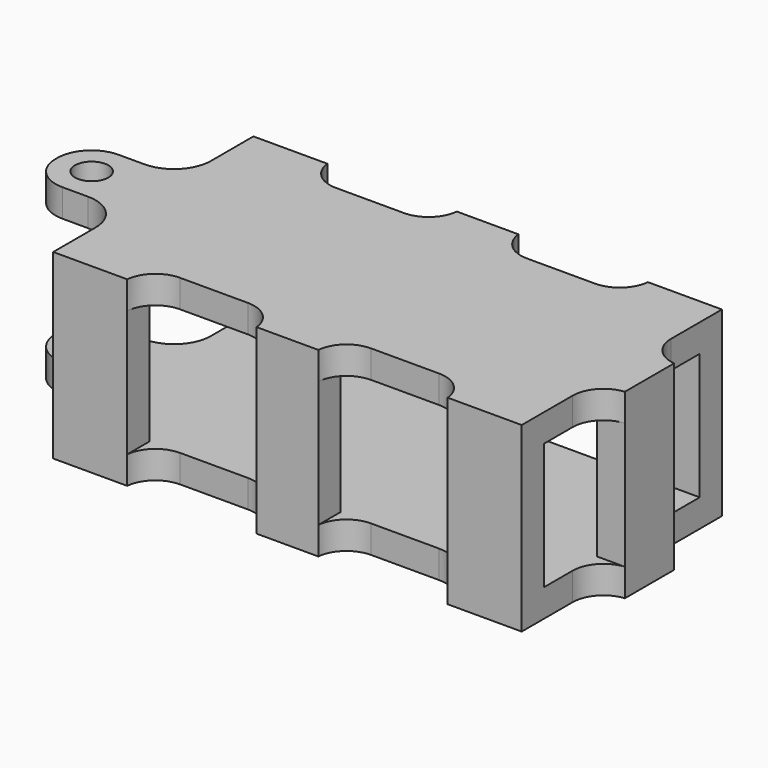
from build123d import *

# Parameters (mm, degrees)
F0_W        = 12
F0_H        = 4.5
F0_W_2      = 4.5
F0_H_2      = 5
F1_DEPTH    = 4.5
F2_DEPTH    = 20.5
F3_START    = 20.5
F3_DEPTH    = 4.5
F4_T1_DEPTH = 4.5
F4_T3_DEPTH = 4.5
F5_T1_DEPTH = 4.5
F5_T3_DEPTH = 4.5
F7_START    = -25
F6_W        = 15.7
F6_H        = 11.4
F6_R        = 2.7
F7_DEPTH    = 4.5
F8_DEPTH    = 4.5
F9_R        = 6
F10_R       = 5.5


# Not quite as in the source:
# - a fillet or chamfer that OpenCascade refuses, or shapes differently, is made with other operations: its cross-section is extruded or revolved along the edge and cut away or added


with BuildPart() as f1:
    # F0 (on Top) → F1 (new body)
    with BuildSketch(Plane.XY):
        Polygon((12, 31.6), (0, 31.6), (0, 0), (12, 0), (33, 0), (38, 0), (43, 0), (64, 0), (76, 0), (76, 10.8), (76, 15.8), (76, 20.8), (76, 31.6), (64, 31.6), (43, 31.6), (38, 31.6), (33, 31.6), align=None)
        with Locations((6, -2.25)):
            Rectangle(F0_W, F0_H)
        Polygon((38, 0), (33, 0), (33, -4.5), (43, -4.5), (43, 0), align=None)
        with Locations((70, -2.25)):
            Rectangle(F0_W, F0_H)
        with Locations((78.25, 13.3)):
            Rectangle(F0_W_2, F0_H_2)
        with Locations((78.25, 18.3)):
            Rectangle(F0_W_2, F0_H_2)
        with Locations((70, 33.85)):
            Rectangle(F0_W, F0_H)
        Polygon((33, 36.1), (33, 31.6), (38, 31.6), (43, 31.6), (43, 36.1), align=None)
        with Locations((6, 33.85)):
            Rectangle(F0_W, F0_H)
    extrude(amount=-F1_DEPTH)

    # F0 (on Top) → F2 (join)
    with BuildSketch(Plane.XY):
        with Locations((6, -2.25)):
            Rectangle(F0_W, F0_H)
        Polygon((38, 0), (33, 0), (33, -4.5), (43, -4.5), (43, 0), align=None)
        Polygon((33, 36.1), (33, 31.6), (38, 31.6), (43, 31.6), (43, 36.1), align=None)
        with Locations((6, 33.85)):
            Rectangle(F0_W, F0_H)
        with Locations((70, -2.25)):
            Rectangle(F0_W, F0_H)
        with Locations((78.25, 13.3)):
            Rectangle(F0_W_2, F0_H_2)
        with Locations((78.25, 18.3)):
            Rectangle(F0_W_2, F0_H_2)
        with Locations((70, 33.85)):
            Rectangle(F0_W, F0_H)
    extrude(amount=F2_DEPTH)

    # F0 (on Top) → F3 (join)
    with BuildSketch(Plane.XY.offset(F3_START)):
        with Locations((6, 33.85)):
            Rectangle(F0_W, F0_H)
        Polygon((12, 31.6), (0, 31.6), (0, 0), (12, 0), (33, 0), (38, 0), (43, 0), (64, 0), (76, 0), (76, 10.8), (76, 15.8), (76, 20.8), (76, 31.6), (64, 31.6), (43, 31.6), (38, 31.6), (33, 31.6), align=None)
        with Locations((6, -2.25)):
            Rectangle(F0_W, F0_H)
        Polygon((33, 36.1), (33, 31.6), (38, 31.6), (43, 31.6), (43, 36.1), align=None)
        Polygon((38, 0), (33, 0), (33, -4.5), (43, -4.5), (43, 0), align=None)
        with Locations((70, 33.85)):
            Rectangle(F0_W, F0_H)
        with Locations((70, -2.25)):
            Rectangle(F0_W, F0_H)
        with Locations((78.25, 18.3)):
            Rectangle(F0_W_2, F0_H_2)
        with Locations((78.25, 13.3)):
            Rectangle(F0_W_2, F0_H_2)
    extrude(amount=F3_DEPTH)

    # F4: fillet of radius 5 on 18 edges, made by hand

    # F4_s2 → F4_t1 (join)
    with BuildSketch(Plane.XY.offset(20.5)):
        with BuildLine():
            ThreePointArc((16.9749371855, 0), (13.6208352193, -1.2919007565), (12, -4.5))
            Line((12, -4.5), (12, 0))
            Line((12, 0), (16.9749371855, 0))
        make_face()
        with BuildLine():
            ThreePointArc((28.0250628145, 0), (31.3791647807, -1.2919007565), (33, -4.5))
            Line((33, -4.5), (33, 0))
            Line((33, 0), (28.0250628145, 0))
        make_face()
        with BuildLine():
            ThreePointArc((43, -4.5), (44.6208352193, -1.2919007565), (47.9749371855, 0))
            Line((47.9749371855, 0), (43, 0))
            Line((43, 0), (43, -4.5))
        make_face()
        with BuildLine():
            ThreePointArc((64, -4.5), (62.3791647807, -1.2919007565), (59.0250628145, 0))
            Line((59.0250628145, 0), (64, 0))
            Line((64, 0), (64, -4.5))
        make_face()
        with BuildLine():
            ThreePointArc((76, 5.8250628145), (77.2919007565, 9.1791647807), (80.5, 10.8))
            Line((80.5, 10.8), (76, 10.8))
            Line((76, 10.8), (76, 5.8250628145))
        make_face()
        with BuildLine():
            ThreePointArc((80.5, 20.8), (77.2919007565, 22.4208352193), (76, 25.7749371855))
            Line((76, 25.7749371855), (76, 20.8))
            Line((76, 20.8), (80.5, 20.8))
        make_face()
        with BuildLine():
            ThreePointArc((43, 36.1), (44.6208352193, 32.8919007565), (47.9749371855, 31.6))
            Line((47.9749371855, 31.6), (43, 31.6))
            Line((43, 31.6), (43, 36.1))
        make_face()
        with BuildLine():
            ThreePointArc((12, 36.1), (13.6208352193, 32.8919007565), (16.9749371855, 31.6))
            Line((16.9749371855, 31.6), (12, 31.6))
            Line((12, 31.6), (12, 36.1))
        make_face()
        with BuildLine():
            ThreePointArc((64, 36.1), (62.3791647807, 32.8919007565), (59.0250628145, 31.6))
            Line((59.0250628145, 31.6), (64, 31.6))
            Line((64, 31.6), (64, 36.1))
        make_face()
    extrude(amount=F4_T1_DEPTH)

    # F4_s4 → F4_t3 (join)
    with BuildSketch(Plane.XY.offset(-4.5)):
        with BuildLine():
            ThreePointArc((16.9749371855, 0), (13.6208352193, -1.2919007565), (12, -4.5))
            Line((12, -4.5), (12, 0))
            Line((12, 0), (16.9749371855, 0))
        make_face()
        with BuildLine():
            ThreePointArc((33, -4.5), (31.3791647807, -1.2919007565), (28.0250628145, 0))
            Line((28.0250628145, 0), (33, 0))
            Line((33, 0), (33, -4.5))
        make_face()
        with BuildLine():
            ThreePointArc((43, -4.5), (44.6208352193, -1.2919007565), (47.9749371855, 0))
            Line((47.9749371855, 0), (43, 0))
            Line((43, 0), (43, -4.5))
        make_face()
        with BuildLine():
            ThreePointArc((59.0250628145, 0), (62.3791647807, -1.2919007565), (64, -4.5))
            Line((64, -4.5), (64, 0))
            Line((64, 0), (59.0250628145, 0))
        make_face()
        with BuildLine():
            ThreePointArc((76, 5.8250628145), (77.2919007565, 9.1791647807), (80.5, 10.8))
            Line((80.5, 10.8), (76, 10.8))
            Line((76, 10.8), (76, 5.8250628145))
        make_face()
        with BuildLine():
            ThreePointArc((80.5, 20.8), (77.2919007565, 22.4208352193), (76, 25.7749371855))
            Line((76, 25.7749371855), (76, 20.8))
            Line((76, 20.8), (80.5, 20.8))
        make_face()
        with BuildLine():
            ThreePointArc((47.9749371855, 31.6), (44.6208352193, 32.8919007565), (43, 36.1))
            Line((43, 36.1), (43, 31.6))
            Line((43, 31.6), (47.9749371855, 31.6))
        make_face()
        with BuildLine():
            ThreePointArc((16.9749371855, 31.6), (13.6208352193, 32.8919007565), (12, 36.1))
            Line((12, 36.1), (12, 31.6))
            Line((12, 31.6), (16.9749371855, 31.6))
        make_face()
        with BuildLine():
            ThreePointArc((64, 36.1), (62.3791647807, 32.8919007565), (59.0250628145, 31.6))
            Line((59.0250628145, 31.6), (64, 31.6))
            Line((64, 31.6), (64, 36.1))
        make_face()
    extrude(amount=F4_T3_DEPTH)

    # F5: fillet of radius 5 on 2 edges, made by hand

    # F5_s2 → F5_t1 (join)
    with BuildSketch(Plane.XY.offset(20.5)):
        with BuildLine():
            ThreePointArc((33, 36.1), (31.3791647807, 32.8919007565), (28.0250628145, 31.6))
            Line((28.0250628145, 31.6), (33, 31.6))
            Line((33, 31.6), (33, 36.1))
        make_face()
    extrude(amount=F5_T1_DEPTH)

    # F5_s4 → F5_t3 (join)
    with BuildSketch(Plane.XY.offset(-4.5)):
        with BuildLine():
            ThreePointArc((33, 36.1), (31.3791647807, 32.8919007565), (28.0250628145, 31.6))
            Line((28.0250628145, 31.6), (33, 31.6))
            Line((33, 31.6), (33, 36.1))
        make_face()
    extrude(amount=F5_T3_DEPTH)

    # F6 (on face) → F7 (join)
    with BuildSketch(Plane.XY.offset(25).offset(F7_START)):
        with Locations((-7.85, 15.8)):
            Rectangle(F6_W, F6_H)
        with Locations((-10, 15.8)):
            Circle(F6_R, mode=Mode.SUBTRACT)
    extrude(amount=-F7_DEPTH)

    # F6 (on face) → F8 (join)
    with BuildSketch(Plane.XY.offset(25)):
        with Locations((-7.85, 15.8)):
            Rectangle(F6_W, F6_H)
        with Locations((-10, 15.8)):
            Circle(F6_R, mode=Mode.SUBTRACT)
    extrude(amount=-F8_DEPTH)

    # F9
    f9_edges = [f1.edges().sort_by_distance(p)[0] for p in [
        (0, 21.5, 22.75),
        (0, 10.1, 22.75),
        (0, 10.1, -2.25),
        (0, 21.5, -2.25),
    ]]
    fillet(f9_edges, radius=F9_R)

    # F10
    f10_edges = [f1.edges().sort_by_distance(p)[0] for p in [
        (-15.7, 21.5, 22.75),
        (-15.7, 10.1, 22.75),
        (-15.7, 10.1, -2.25),
        (-15.7, 21.5, -2.25),
    ]]
    fillet(f10_edges, radius=F10_R)


solid = f1.part
